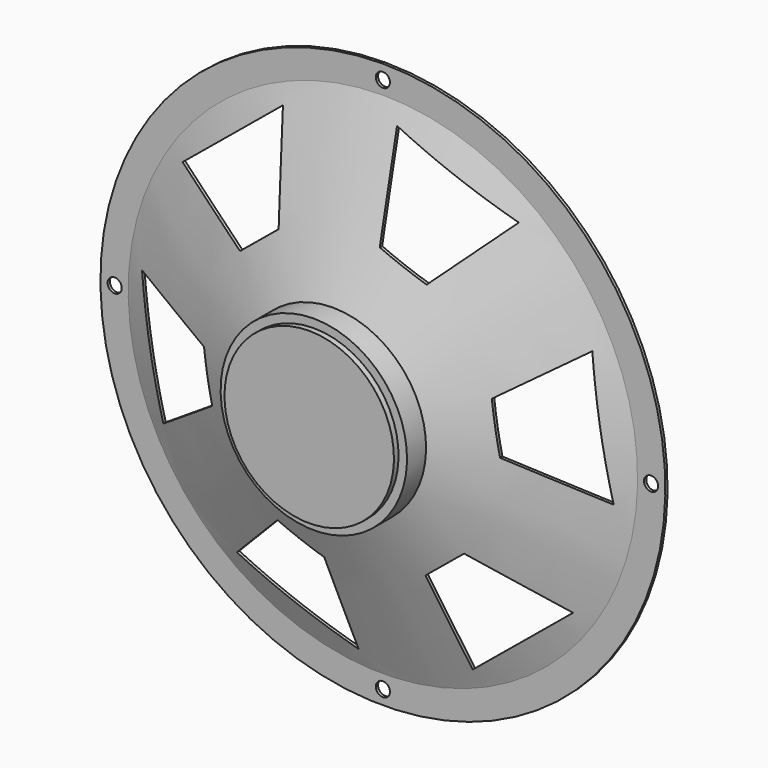
from build123d import *

# Parameters (mm, degrees)
F0_W          = 2.0318743463
F0_H          = 30
F0_W_2        = 1.8593237499
F2_W          = 8.4245346444
F2_H          = 33
F9_DEPTH      = 135
F9_DEPTH_BACK = 304
F10_COUNT     = 6
F12_R         = 2.5
F13_DEPTH     = 33.5917390977


# Not quite as in the source:
# - the program builds the solid bodies; features that only make, move or delete a surface that nothing else refers to are left out


with BuildPart() as f1:
    # F0 (on Right) → F1 (revolve)
    with BuildSketch(Plane.YZ):
        with Locations((1.0159371731, 15)):
            Rectangle(F0_W, F0_H)
    revolve(axis=Axis((0, 1.0159371731, 0), (0, 1, 0)))


with BuildPart() as f1b:
    # F0 (on Right) → F1, piece 2 (revolve)
    with BuildSketch(Plane.YZ):
        with Locations((11.3860708656, 15)):
            Rectangle(F0_W_2, F0_H)
    revolve(axis=Axis((0, 1.0159371731, 0), (0, 1, 0)))


with BuildPart() as f3:
    # F2 (on Right) → F3 (revolve)
    with BuildSketch(Plane.YZ):
        with Locations((6.2441416685, 16.5)):
            Rectangle(F2_W, F2_H)
    revolve(axis=Axis((0, 6.2441416685, 0), (0, 1, 0)))


with BuildPart() as f7:
    # F6 (on Right) → F7 (revolve)
    with BuildSketch(Plane.YZ):
        Polygon((0, 0), (1.0633068526, 0), (33.5907390977, 90), (33.5907390977, 100), (32.5907390977, 100), (32.5907390977, 90.1751634341), align=None)
    revolve(axis=Axis((0, 47.4777109921, 0), (0, 1, 0)))


with BuildPart() as f9:
    # F8 (on Front) → F9 (new body, two sides)
    with BuildSketch(Plane.XZ) as f9_sk:
        Polygon((-33.5954686136, 77.0091775446), (-69.1209128956, 47.7636717384), (-39.6688894061, 34.2418646839), (-25.9834363433, 45.5080994937), align=None)
    extrude(amount=F9_DEPTH)
    extrude(f9_sk.sketch, amount=-F9_DEPTH_BACK)


with BuildPart() as f10_1:
    # F10: instance of F9
    add(f9.part.rotate(Axis((0, 11.3860708656, 0), (0, 1, 0)), 1 * 360 / F10_COUNT))


with BuildPart() as f10_2:
    # F10: instance of F9
    add(f9.part.rotate(Axis((0, 11.3860708656, 0), (0, 1, 0)), 2 * 360 / F10_COUNT))


with BuildPart() as f10_3:
    # F10: instance of F9
    add(f9.part.rotate(Axis((0, 11.3860708656, 0), (0, 1, 0)), 3 * 360 / F10_COUNT))


with BuildPart() as f10_4:
    # F10: instance of F9
    add(f9.part.rotate(Axis((0, 11.3860708656, 0), (0, 1, 0)), 4 * 360 / F10_COUNT))


with BuildPart() as f10_5:
    # F10: instance of F9
    add(f9.part.rotate(Axis((0, 11.3860708656, 0), (0, 1, 0)), 5 * 360 / F10_COUNT))


with BuildPart() as f7_1:
    add(f7.part)

    # F11: cut F10_1, F9, F10_5, F10_4, F10_3, F10_2
    add(f10_1.part, mode=Mode.SUBTRACT)
    add(f9.part, mode=Mode.SUBTRACT)
    add(f10_5.part, mode=Mode.SUBTRACT)
    add(f10_4.part, mode=Mode.SUBTRACT)
    add(f10_3.part, mode=Mode.SUBTRACT)
    add(f10_2.part, mode=Mode.SUBTRACT)

    # F12 (on face) → F13 (cut, through all)
    with BuildSketch(Plane(origin=(0, 33.5907390977, 0), x_dir=(-1, 0, 0), z_dir=(0, 1, 0))):
        with Locations((94.9471559662, 0)):
            Circle(F12_R)
        with Locations((-94.9471559662, 0)):
            Circle(F12_R)
        with Locations((0, -94.9471559662)):
            Circle(F12_R)
        with Locations((0, 94.9471559662)):
            Circle(F12_R)
    extrude(amount=-F13_DEPTH, mode=Mode.SUBTRACT)


solid = Compound([f1.part, f1b.part, f3.part, f7_1.part])
